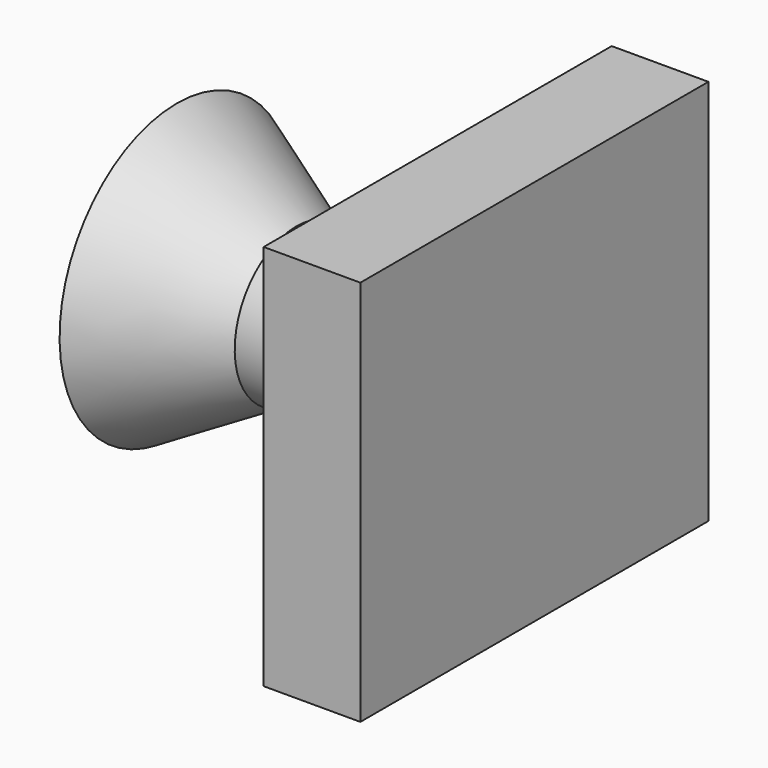
from build123d import *

# Parameters (mm, degrees)
F2_T            = 2.54
F3_R            = 2.54
F4_DEPTH        = 25.4
F4_COPIES_COUNT = 8
F5_R            = 2.54
F6_DEPTH        = 25.4
F8_W            = 114.3
F8_H            = 101.6
F9_DEPTH        = 25.4
F10_T           = -2.54


# Not quite as in the source:
# - a pattern or mirror of a feature is missing from the dataset's text; its kind, count and spacing are read off the source's solid


with BuildPart() as f1:
    # F0 (on Front) → F1 (revolve)
    with BuildSketch(Plane.XZ):
        Polygon((-25.0586248056, 17.78), (-55.8544881642, 35.56), (-55.8544881642, 0), (25.7413751944, 0), (25.7413751944, 17.78), align=None)
    revolve(axis=Axis((-15.0565564849, 0, 0), (-1, 0, 0)))

    # F2
    f2_openings = [f1.faces().sort_by_distance(p)[0] for p in [
        (-55.854488, 0, 0),
    ]]
    offset(amount=F2_T, openings=f2_openings, kind=Kind.INTERSECTION)

    # F3 (on face) → F4 (cut)
    with BuildSketch(Plane.YZ.offset(28.2813751944)):
        with Locations((-7.6700180371, 11.6761176472)):
            Circle(F3_R)
    f4 = extrude(amount=-F4_DEPTH, mode=Mode.SUBTRACT)

    # F4_copies: F4 ×8 about axis
    f4_copies_axis = Axis((0, 0, 0), (1, 0, 0))
    for i in range(1, F4_COPIES_COUNT):
        add(f4.rotate(f4_copies_axis, i * 360 / F4_COPIES_COUNT), mode=Mode.SUBTRACT)

    # F5 (on face) → F6 (cut)
    with BuildSketch(Plane.YZ.offset(28.2813751944)):
        Circle(F5_R)
    extrude(amount=-F6_DEPTH, mode=Mode.SUBTRACT)


with BuildPart() as f9:
    # F8 (on offset) → F9 (new body)
    with BuildSketch(Plane.YZ.offset(12.7)):
        Rectangle(F8_W, F8_H)
    extrude(amount=F9_DEPTH)

    # F10
    f10_openings = [f9.faces().sort_by_distance(p)[0] for p in [
        (12.7, 0, 0),
    ]]
    offset(amount=F10_T, openings=f10_openings)


solid = Compound([f1.part, f9.part])
